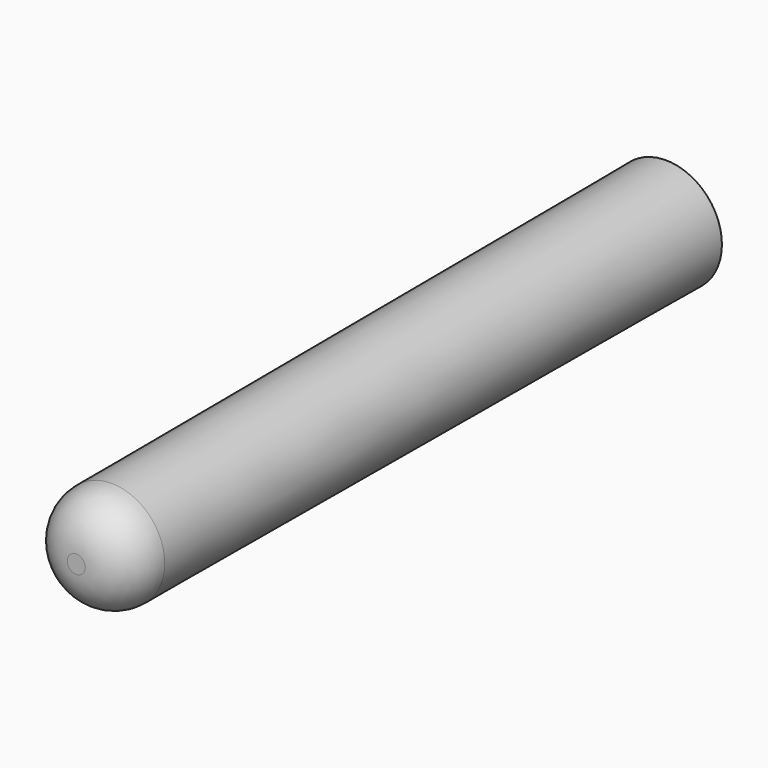
from build123d import *

# Parameters (mm, degrees)
F0_R = 19
F2_R = 18
F4_R = 15


with BuildPart() as f3:
    # F0 (on Front) → F3 section 0
    with BuildSketch(Plane.XZ):
        Circle(F0_R)
    # F2 (on offset) → F3 section 1
    with BuildSketch(Plane.XZ.offset(250)):
        Circle(F2_R)
    loft()

    # F4
    f4_edges = [f3.edges().sort_by_distance(p)[0] for p in [
        (-18, -250, 0),
    ]]
    fillet(f4_edges, radius=F4_R)


solid = f3.part
